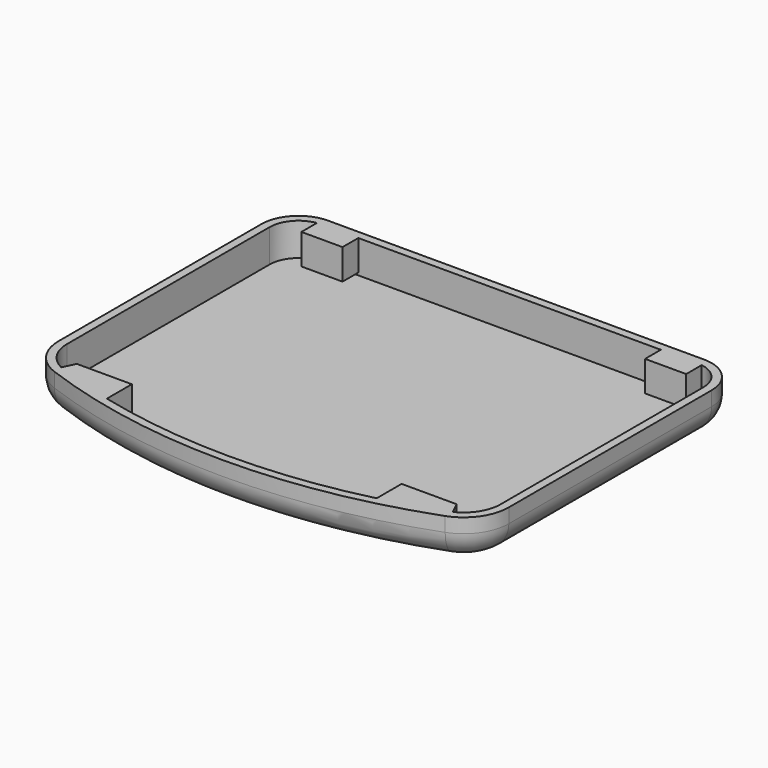
from build123d import *

# Parameters (mm, degrees)
F1_DEPTH = 12.7
F2_T     = -2.54
F3_R     = 8.255
F5_W     = 12.7
F5_H     = 6.35
F6_DEPTH = 9.398


# Not quite as in the source:
# - a feature names something its author has since deleted; it is built from what else it names


with BuildPart() as f1:
    # F0 (on Top) → F1 (new body)
    with BuildSketch(Plane.XY):
        with BuildLine():
            Line((58.0965084505, 62.5356453779), (-58.0965084505, 62.5356453779))
            ThreePointArc((-58.0965084505, 62.5356453779), (-66.1787389595, 59.1878758868), (-69.5265084505, 51.1056453779))
            Line((-69.5265084505, 51.1056453779), (-69.5265084505, -27.1992570698))
            ThreePointArc((-69.5265084505, -27.1992570698), (-67.0115325937, -35.1957139026), (-60.3721316603, -40.3130159932))
            ThreePointArc((-60.3721316603, -40.3130159932), (0, -51.0474727306), (60.3721316603, -40.3130159932))
            ThreePointArc((60.3721316603, -40.3130159932), (67.0115325937, -35.1957139026), (69.5265084505, -27.1992570698))
            Line((69.5265084505, -27.1992570698), (69.5265084505, 51.1056453779))
            ThreePointArc((69.5265084505, 51.1056453779), (66.1787389595, 59.1878758868), (58.0965084505, 62.5356453779))
        make_face()
    extrude(amount=F1_DEPTH)

    # F2
    f2_openings = [f1.faces().sort_by_distance(p)[0] for p in [
        (0, 7.919531, 12.7),
    ]]
    offset(amount=F2_T, openings=f2_openings)

    # F3
    f3_edges = [f1.edges().sort_by_distance(p)[0] for p in [
        (69.526508, 11.953194, 0),
        (66.178739, 59.187876, 0),
        (0, 62.535645, 0),
        (-66.178739, 59.187876, 0),
        (-69.526508, 11.953194, 0),
        (-67.011533, -35.195714, 0),
        (0, -51.047473, 0),
        (67.011533, -35.195714, 0),
    ]]
    fillet(f3_edges, radius=F3_R)

    # F5 (on offset) → F6 (join)
    with BuildSketch(Plane.XY.offset(12.7)):
        with Locations((-53.0805146158, 57.0815077901)):
            Rectangle(F5_W, F5_H)
        with Locations((53.0805146158, 57.0815077901)):
            Rectangle(F5_W, F5_H)
        Polygon((-41.6677072644, -33.773638308), (-58.6946308613, -33.773638308), (-60.6418885291, -37.9110425711), (-53.9016760886, -40.266495198), (-41.6677072644, -43.4330925345), align=None)
        Polygon((60.6418885291, -37.9110425711), (58.6946308613, -33.773638308), (41.6677072644, -33.773638308), (41.6677072644, -43.4330925345), (53.9016760886, -40.266495198), align=None)
    extrude(amount=-F6_DEPTH)


solid = f1.part
